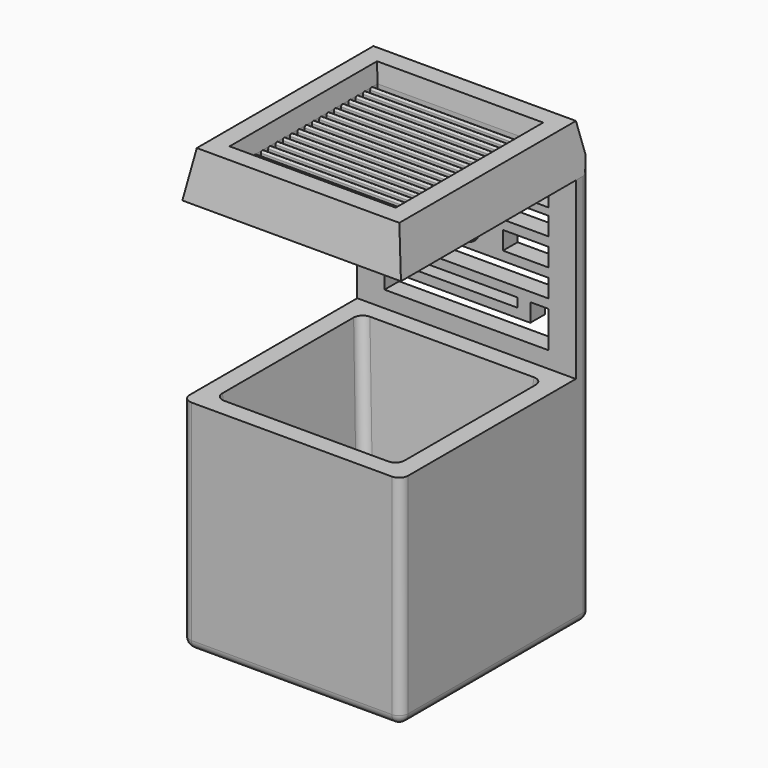
from build123d import *

# Parameters (mm, degrees)
F1_W                    = 120
F1_H                    = 120
F2_DEPTH                = 120
F4_W                    = 100
F4_H                    = 100
F5_DEPTH                = 100
DRAFT_F5_DRAFTED_ANGLE  = 5
F3_W                    = 120
F3_H                    = 120
F3_H_2                  = 96
F6_DEPTH                = 10
F7_W                    = 28
F7_H                    = 5
F7_W_2                  = 45
F7_H_2                  = 10
F7_W_3                  = 25
F7_W_4                  = 10
F7_H_3                  = 13
F8_DEPTH                = 10
F9_W                    = 120
F9_H                    = 130
F10_DEPTH               = 25
F10_TAPER               = 10
F11_W                   = 91.1836509646
F11_H                   = 101.1836509646
F12_DEPTH               = 10
DRAFT_F12_DRAFTED_ANGLE = 7
F13_W                   = 88.7279597465
F13_H                   = 3
F14_DEPTH               = 15
F15_T1_DEPTH            = 88.7279597465
F16_R                   = 5
F17_R                   = 5
F17_R_2                 = 2
F17_R_3                 = 3.5
F18_DEPTH               = 20
F18_TAPER               = 3


# Not quite as in the source:
# - a fillet or chamfer that OpenCascade refuses, or shapes differently, is made with other operations: its cross-section is extruded or revolved along the edge and cut away or added
# - an extrude with a draft is written as a straight extrude whose walls are then drafted


with BuildPart() as f2:
    # F1 (on Top) → F2 (new body)
    with BuildSketch(Plane.XY):
        Rectangle(F1_W, F1_H)
    extrude(amount=F2_DEPTH)


with BuildPart() as f5_drafted:
    # F4 (on face) → F5 (new body)
    with BuildSketch(Plane.XY.offset(120)):
        Rectangle(F4_W, F4_H)
    extrude(amount=-F5_DEPTH)

    # draft_F5_drafted
    draft_f5_drafted_walls = [f5_drafted.faces().sort_by_distance(p)[0] for p in [
        (50, 0, 53.3333333333),
        (0, 50, 53.3333333333),
        (-50, 0, 53.3333333333),
        (0, -50, 53.3333333333),
    ]]
    draft(draft_f5_drafted_walls, neutral_plane=Plane(origin=(0, 0, 120), x_dir=(1, 0, 0), z_dir=(0, 0, -1)), angle=DRAFT_F5_DRAFTED_ANGLE)


with BuildPart() as f2_1:
    add(f2.part)

    # join_F5_drafted: cut F5_drafted
    add(f5_drafted.part, mode=Mode.SUBTRACT)

    # F3 (on face) → F6 (join)
    with BuildSketch(Plane(origin=(0, 60, 0), x_dir=(-1, 0, 0), z_dir=(0, 1, 0))):
        with Locations((0, 60)):
            Rectangle(F3_W, F3_H)
        with Locations((0, 168)):
            Rectangle(F3_W, F3_H_2)
    extrude(amount=F6_DEPTH)

    # F7 (on face) → F8 (cut, through all)
    with BuildSketch(Plane.XZ.offset(-60)):
        Polygon((-35, 149), (-45, 149), (-45, 129), (-35, 129), (0, 129), (0, 139), (-35, 139), align=None)
        with Locations((-14, 146.5)):
            Rectangle(F7_W, F7_H)
        Polygon((35, 139), (0, 139), (0, 129), (35, 129), (45, 129), (45, 149), (35, 149), align=None)
        with Locations((14, 146.5)):
            Rectangle(F7_W, F7_H)
        with Locations((-22.5, 159)):
            Rectangle(F7_W_2, F7_H_2)
        with Locations((-32.5, 174)):
            Rectangle(F7_W_3, F7_H_2)
        with Locations((-22.5, 189)):
            Rectangle(F7_W_2, F7_H_2)
        with Locations((-40, 204.5)):
            Rectangle(F7_W_4, F7_H_3)
        with Locations((-12.5, 204.5)):
            Rectangle(F7_W_3, F7_H_3)
        with Locations((12.5, 204.5)):
            Rectangle(F7_W_3, F7_H_3)
        with Locations((40, 204.5)):
            Rectangle(F7_W_4, F7_H_3)
        with Locations((22.5, 189)):
            Rectangle(F7_W_2, F7_H_2)
        with Locations((32.5, 174)):
            Rectangle(F7_W_3, F7_H_2)
        with BuildLine():
            ThreePointArc((0, 167.0751091007), (6.9248908993, 174), (0, 180.9248908993))
            ThreePointArc((0, 180.9248908993), (-6.9248908993, 174), (0, 167.0751091007))
        make_face()
        with Locations((22.5, 159)):
            Rectangle(F7_W_2, F7_H_2)
    extrude(amount=-F8_DEPTH, mode=Mode.SUBTRACT)

    # F9 (on face) → F10 (join)
    with BuildSketch(Plane.XY.offset(216)):
        with Locations((0, 5)):
            Rectangle(F9_W, F9_H)
    extrude(amount=F10_DEPTH, taper=F10_TAPER)


with BuildPart() as f12_drafted:
    # F11 (on face) → F12 (new body)
    with BuildSketch(Plane.XY.offset(241)):
        with Locations((0, 5)):
            Rectangle(F11_W, F11_H)
    extrude(amount=-F12_DEPTH)

    # draft_F12_drafted
    draft_f12_drafted_walls = [f12_drafted.faces().sort_by_distance(p)[0] for p in [
        (45.5918254823, 5, 234.3333333333),
        (0, 55.5918254823, 234.3333333333),
        (-45.5918254823, 5, 234.3333333333),
        (0, -45.5918254823, 234.3333333333),
    ]]
    draft(draft_f12_drafted_walls, neutral_plane=Plane(origin=(0, 0, 241), x_dir=(1, 0, 0), z_dir=(0, 0, -1)), angle=DRAFT_F12_DRAFTED_ANGLE)


with BuildPart() as f2_2:
    add(f2_1.part)

    # join_F12_drafted: cut F12_drafted
    add(f12_drafted.part, mode=Mode.SUBTRACT)

    # F13 (on face) → F14 (cut, through all)
    with BuildSketch(Plane.XY.offset(231)):
        with Locations((0, 52.8639798733)):
            Rectangle(F13_W, F13_H)
        with Locations((0, 47.8639798733)):
            Rectangle(F13_W, F13_H)
        with Locations((0, 42.8639798733)):
            Rectangle(F13_W, F13_H)
        with Locations((0, 37.8639798733)):
            Rectangle(F13_W, F13_H)
        with Locations((0, 32.8639798733)):
            Rectangle(F13_W, F13_H)
        with Locations((0, 27.8639798733)):
            Rectangle(F13_W, F13_H)
        with Locations((0, 22.8639798733)):
            Rectangle(F13_W, F13_H)
        with Locations((0, 17.8639798733)):
            Rectangle(F13_W, F13_H)
        with Locations((0, 12.8639798733)):
            Rectangle(F13_W, F13_H)
        with Locations((0, 7.8639798733)):
            Rectangle(F13_W, F13_H)
        with Locations((0, 2.8639798733)):
            Rectangle(F13_W, F13_H)
        with Locations((0, -2.1360201267)):
            Rectangle(F13_W, F13_H)
        with Locations((0, -7.1360201267)):
            Rectangle(F13_W, F13_H)
        with Locations((0, -12.1360201267)):
            Rectangle(F13_W, F13_H)
        with Locations((0, -17.1360201267)):
            Rectangle(F13_W, F13_H)
        with Locations((0, -22.1360201267)):
            Rectangle(F13_W, F13_H)
        with Locations((0, -27.1360201267)):
            Rectangle(F13_W, F13_H)
        with Locations((0, -32.1360201267)):
            Rectangle(F13_W, F13_H)
        with Locations((0, -37.1360201267)):
            Rectangle(F13_W, F13_H)
        with Locations((0, -42.1360201267)):
            Rectangle(F13_W, F13_H)
    extrude(amount=-F14_DEPTH, mode=Mode.SUBTRACT)

    # F15: fillet of radius 1 on 39 edges, made by hand

    # F15_s2 → F15_t1 (cut)
    with BuildSketch(Plane.YZ.offset(-44.3639798733)):
        with BuildLine():
            ThreePointArc((51.3639798733, 230), (51.0710866544, 230.7071067812), (50.3639798733, 231))
            Line((50.3639798733, 231), (51.3639798733, 231))
            Line((51.3639798733, 231), (51.3639798733, 230))
        make_face()
        with BuildLine():
            ThreePointArc((49.3639798733, 230), (49.6568730921, 230.7071067812), (50.3639798733, 231))
            Line((50.3639798733, 231), (49.3639798733, 231))
            Line((49.3639798733, 231), (49.3639798733, 230))
        make_face()
        with BuildLine():
            ThreePointArc((46.3639798733, 230), (46.0710866544, 230.7071067812), (45.3639798733, 231))
            Line((45.3639798733, 231), (46.3639798733, 231))
            Line((46.3639798733, 231), (46.3639798733, 230))
        make_face()
        with BuildLine():
            ThreePointArc((44.3639798733, 230), (44.6568730921, 230.7071067812), (45.3639798733, 231))
            Line((45.3639798733, 231), (44.3639798733, 231))
            Line((44.3639798733, 231), (44.3639798733, 230))
        make_face()
        with BuildLine():
            ThreePointArc((41.3639798733, 230), (41.0710866544, 230.7071067812), (40.3639798733, 231))
            Line((40.3639798733, 231), (41.3639798733, 231))
            Line((41.3639798733, 231), (41.3639798733, 230))
        make_face()
        with BuildLine():
            ThreePointArc((39.3639798733, 230), (39.6568730921, 230.7071067812), (40.3639798733, 231))
            Line((40.3639798733, 231), (39.3639798733, 231))
            Line((39.3639798733, 231), (39.3639798733, 230))
        make_face()
        with BuildLine():
            ThreePointArc((36.3639798733, 230), (36.0710866544, 230.7071067812), (35.3639798733, 231))
            Line((35.3639798733, 231), (36.3639798733, 231))
            Line((36.3639798733, 231), (36.3639798733, 230))
        make_face()
        with BuildLine():
            ThreePointArc((34.3639798733, 230), (34.6568730921, 230.7071067812), (35.3639798733, 231))
            Line((35.3639798733, 231), (34.3639798733, 231))
            Line((34.3639798733, 231), (34.3639798733, 230))
        make_face()
        with BuildLine():
            ThreePointArc((31.3639798733, 230), (31.0710866544, 230.7071067812), (30.3639798733, 231))
            Line((30.3639798733, 231), (31.3639798733, 231))
            Line((31.3639798733, 231), (31.3639798733, 230))
        make_face()
        with BuildLine():
            ThreePointArc((29.3639798733, 230), (29.6568730921, 230.7071067812), (30.3639798733, 231))
            Line((30.3639798733, 231), (29.3639798733, 231))
            Line((29.3639798733, 231), (29.3639798733, 230))
        make_face()
        with BuildLine():
            ThreePointArc((26.3639798733, 230), (26.0710866544, 230.7071067812), (25.3639798733, 231))
            Line((25.3639798733, 231), (26.3639798733, 231))
            Line((26.3639798733, 231), (26.3639798733, 230))
        make_face()
        with BuildLine():
            ThreePointArc((24.3639798733, 230), (24.6568730921, 230.7071067812), (25.3639798733, 231))
            Line((25.3639798733, 231), (24.3639798733, 231))
            Line((24.3639798733, 231), (24.3639798733, 230))
        make_face()
        with BuildLine():
            ThreePointArc((21.3639798733, 230), (21.0710866544, 230.7071067812), (20.3639798733, 231))
            Line((20.3639798733, 231), (21.3639798733, 231))
            Line((21.3639798733, 231), (21.3639798733, 230))
        make_face()
        with BuildLine():
            ThreePointArc((19.3639798733, 230), (19.6568730921, 230.7071067812), (20.3639798733, 231))
            Line((20.3639798733, 231), (19.3639798733, 231))
            Line((19.3639798733, 231), (19.3639798733, 230))
        make_face()
        with BuildLine():
            ThreePointArc((16.3639798733, 230), (16.0710866544, 230.7071067812), (15.3639798733, 231))
            Line((15.3639798733, 231), (16.3639798733, 231))
            Line((16.3639798733, 231), (16.3639798733, 230))
        make_face()
        with BuildLine():
            ThreePointArc((14.3639798733, 230), (14.6568730921, 230.7071067812), (15.3639798733, 231))
            Line((15.3639798733, 231), (14.3639798733, 231))
            Line((14.3639798733, 231), (14.3639798733, 230))
        make_face()
        with BuildLine():
            ThreePointArc((11.3639798733, 230), (11.0710866544, 230.7071067812), (10.3639798733, 231))
            Line((10.3639798733, 231), (11.3639798733, 231))
            Line((11.3639798733, 231), (11.3639798733, 230))
        make_face()
        with BuildLine():
            ThreePointArc((9.3639798733, 230), (9.6568730921, 230.7071067812), (10.3639798733, 231))
            Line((10.3639798733, 231), (9.3639798733, 231))
            Line((9.3639798733, 231), (9.3639798733, 230))
        make_face()
        with BuildLine():
            ThreePointArc((-5.6360201267, 230), (-5.3431269079, 230.7071067812), (-4.6360201267, 231))
            Line((-4.6360201267, 231), (-5.6360201267, 231))
            Line((-5.6360201267, 231), (-5.6360201267, 230))
        make_face()
        with BuildLine():
            ThreePointArc((-8.6360201267, 230), (-8.9289133456, 230.7071067812), (-9.6360201267, 231))
            Line((-9.6360201267, 231), (-8.6360201267, 231))
            Line((-8.6360201267, 231), (-8.6360201267, 230))
        make_face()
        with BuildLine():
            ThreePointArc((-10.6360201267, 230), (-10.3431269079, 230.7071067812), (-9.6360201267, 231))
            Line((-9.6360201267, 231), (-10.6360201267, 231))
            Line((-10.6360201267, 231), (-10.6360201267, 230))
        make_face()
        with BuildLine():
            ThreePointArc((-13.6360201267, 230), (-13.9289133456, 230.7071067812), (-14.6360201267, 231))
            Line((-14.6360201267, 231), (-13.6360201267, 231))
            Line((-13.6360201267, 231), (-13.6360201267, 230))
        make_face()
        with BuildLine():
            ThreePointArc((-15.6360201267, 230), (-15.3431269079, 230.7071067812), (-14.6360201267, 231))
            Line((-14.6360201267, 231), (-15.6360201267, 231))
            Line((-15.6360201267, 231), (-15.6360201267, 230))
        make_face()
        with BuildLine():
            ThreePointArc((-18.6360201267, 230), (-18.9289133456, 230.7071067812), (-19.6360201267, 231))
            Line((-19.6360201267, 231), (-18.6360201267, 231))
            Line((-18.6360201267, 231), (-18.6360201267, 230))
        make_face()
        with BuildLine():
            ThreePointArc((-20.6360201267, 230), (-20.3431269079, 230.7071067812), (-19.6360201267, 231))
            Line((-19.6360201267, 231), (-20.6360201267, 231))
            Line((-20.6360201267, 231), (-20.6360201267, 230))
        make_face()
        with BuildLine():
            ThreePointArc((-23.6360201267, 230), (-23.9289133456, 230.7071067812), (-24.6360201267, 231))
            Line((-24.6360201267, 231), (-23.6360201267, 231))
            Line((-23.6360201267, 231), (-23.6360201267, 230))
        make_face()
        with BuildLine():
            ThreePointArc((-25.6360201267, 230), (-25.3431269079, 230.7071067812), (-24.6360201267, 231))
            Line((-24.6360201267, 231), (-25.6360201267, 231))
            Line((-25.6360201267, 231), (-25.6360201267, 230))
        make_face()
        with BuildLine():
            ThreePointArc((-28.6360201267, 230), (-28.9289133456, 230.7071067812), (-29.6360201267, 231))
            Line((-29.6360201267, 231), (-28.6360201267, 231))
            Line((-28.6360201267, 231), (-28.6360201267, 230))
        make_face()
        with BuildLine():
            ThreePointArc((-30.6360201267, 230), (-30.3431269079, 230.7071067812), (-29.6360201267, 231))
            Line((-29.6360201267, 231), (-30.6360201267, 231))
            Line((-30.6360201267, 231), (-30.6360201267, 230))
        make_face()
        with BuildLine():
            ThreePointArc((-3.6360201267, 230), (-3.9289133456, 230.7071067812), (-4.6360201267, 231))
            Line((-4.6360201267, 231), (-3.6360201267, 231))
            Line((-3.6360201267, 231), (-3.6360201267, 230))
        make_face()
        with BuildLine():
            ThreePointArc((-0.6360201267, 230), (-0.3431269079, 230.7071067812), (0.3639798733, 231))
            Line((0.3639798733, 231), (-0.6360201267, 231))
            Line((-0.6360201267, 231), (-0.6360201267, 230))
        make_face()
        with BuildLine():
            ThreePointArc((1.3639798733, 230), (1.0710866544, 230.7071067812), (0.3639798733, 231))
            Line((0.3639798733, 231), (1.3639798733, 231))
            Line((1.3639798733, 231), (1.3639798733, 230))
        make_face()
        with BuildLine():
            ThreePointArc((4.3639798733, 230), (4.6568730921, 230.7071067812), (5.3639798733, 231))
            Line((5.3639798733, 231), (4.3639798733, 231))
            Line((4.3639798733, 231), (4.3639798733, 230))
        make_face()
        with BuildLine():
            ThreePointArc((6.3639798733, 230), (6.0710866544, 230.7071067812), (5.3639798733, 231))
            Line((5.3639798733, 231), (6.3639798733, 231))
            Line((6.3639798733, 231), (6.3639798733, 230))
        make_face()
        with BuildLine():
            ThreePointArc((-35.6360201267, 230), (-35.3431269079, 230.7071067812), (-34.6360201267, 231))
            Line((-34.6360201267, 231), (-35.6360201267, 231))
            Line((-35.6360201267, 231), (-35.6360201267, 230))
        make_face()
        with BuildLine():
            ThreePointArc((-33.6360201267, 230), (-33.9289133456, 230.7071067812), (-34.6360201267, 231))
            Line((-34.6360201267, 231), (-33.6360201267, 231))
            Line((-33.6360201267, 231), (-33.6360201267, 230))
        make_face()
        with BuildLine():
            ThreePointArc((-40.6360201267, 230), (-40.3431269079, 230.7071067812), (-39.6360201267, 231))
            Line((-39.6360201267, 231), (-40.6360201267, 231))
            Line((-40.6360201267, 231), (-40.6360201267, 230))
        make_face()
        with BuildLine():
            ThreePointArc((-38.6360201267, 230), (-38.9289133456, 230.7071067812), (-39.6360201267, 231))
            Line((-39.6360201267, 231), (-38.6360201267, 231))
            Line((-38.6360201267, 231), (-38.6360201267, 230))
        make_face()
        with BuildLine():
            ThreePointArc((-43.6360201267, 230.0377141275), (-43.8385114266, 230.6410215725), (-44.3639798733, 231))
            Line((-44.3639798733, 231), (-43.6360201267, 231))
            Line((-43.6360201267, 231), (-43.6360201267, 230.0377141275))
        make_face()
    extrude(amount=F15_T1_DEPTH, mode=Mode.SUBTRACT)

    # F16
    f16_edges = [f2_2.edges().sort_by_distance(p)[0] for p in [
        (0, -60, 0),
        (-60, 5, 0),
        (60, 5, 0),
        (0, 70, 0),
        (60, 70, 108),
        (60, -60, 60),
        (-60, -60, 60),
        (-60, 70, 108),
        (-45.625567, -45.625567, 70),
        (45.625567, -45.625567, 70),
        (0, -41.251134, 20),
        (41.251134, 0, 20),
        (0, 41.251134, 20),
        (-41.251134, 0, 20),
        (-45.625567, 45.625567, 70),
        (45.625567, 45.625567, 70),
    ]]
    fillet(f16_edges, radius=F16_R)

    # F17 (on face) → F18 (cut, through all)
    with BuildSketch(Plane(origin=(0, 0, 0), x_dir=(1, 0, 0), z_dir=(0, 0, -1))):
        Circle(F17_R)
        with Locations((0, 11)):
            Circle(F17_R_2)
        with Locations((0, 21)):
            Circle(F17_R_3)
        with Locations((-11.3534571666, 17.6663241895)):
            Circle(F17_R_3)
        with Locations((-19.1022719024, 8.723715273)):
            Circle(F17_R_3)
        with Locations((-20.7862502795, -2.9886116037)):
            Circle(F17_R_3)
        with Locations((-15.8707410614, -13.7520754129)):
            Circle(F17_R_3)
        with Locations((-5.9163836937, -20.1493524459)):
            Circle(F17_R_3)
        with Locations((5.9163836937, -20.1493524459)):
            Circle(F17_R_3)
        with Locations((-8.6001463071, 6.8583878204)):
            Circle(F17_R_2)
        with Locations((-10.724207034, -2.4477302735)):
            Circle(F17_R_2)
        with Locations((-4.7727211303, -9.9106575469)):
            Circle(F17_R_2)
        with Locations((4.7727211303, -9.9106575469)):
            Circle(F17_R_2)
        with Locations((10.724207034, -2.4477302735)):
            Circle(F17_R_2)
        with Locations((8.6001463071, 6.8583878204)):
            Circle(F17_R_2)
        with Locations((15.8707410614, -13.7520754129)):
            Circle(F17_R_3)
        with Locations((20.7862502795, -2.9886116037)):
            Circle(F17_R_3)
        with Locations((19.1022719024, 8.723715273)):
            Circle(F17_R_3)
        with Locations((11.3534571666, 17.6663241895)):
            Circle(F17_R_3)
    extrude(amount=-F18_DEPTH, taper=F18_TAPER, mode=Mode.SUBTRACT)


solid = f2_2.part
